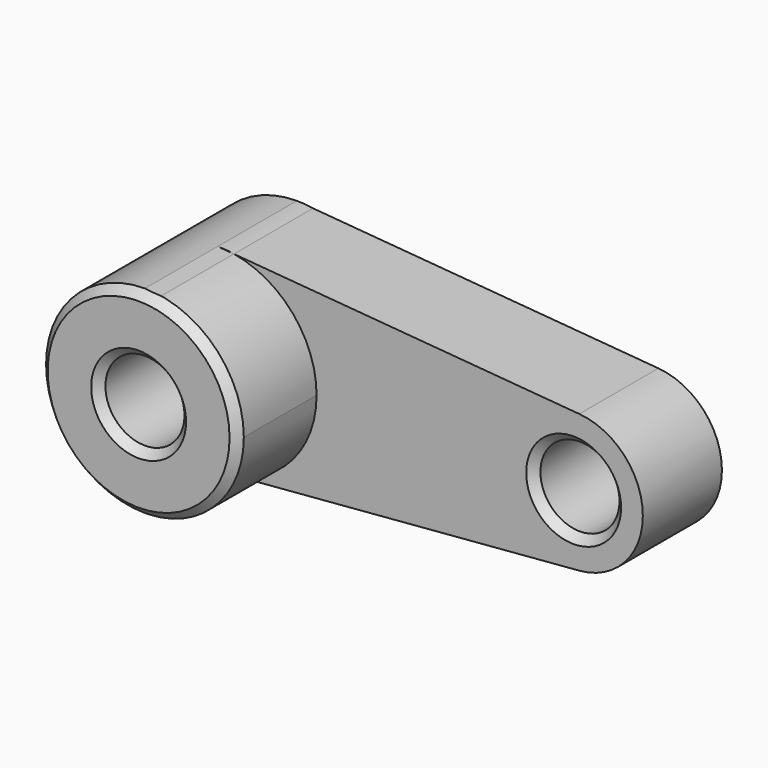
from build123d import *

# Parameters (mm, degrees)
F0_R        = 10
F1_DEPTH    = 25
F2_DEPTH    = 25
F3_T2_ANGLE = 203.6133668192
F3_T8_ANGLE = 184.7022290241


# Not quite as in the source:
# - a fillet or chamfer that OpenCascade refuses, or shapes differently, is made with other operations: its cross-section is extruded or revolved along the edge and cut away or added


with BuildPart() as f1:
    # F0 (on Front) → F1 (new body)
    with BuildSketch(Plane.XZ):
        with BuildLine():
            Line((4.1054428346, 24.6606029758), (0, 25))
            ThreePointArc((0, 25), (-25, 0), (0, -25))
            Line((0, -25), (4.1054428346, -24.6606029758))
            ThreePointArc((4.1054428346, -24.6606029758), (19.0740146648, -16.1611251022), (25, 0))
            ThreePointArc((25, 0), (19.0740146648, 16.1611251022), (4.1054428346, 24.6606029758))
        make_face()
        Circle(F0_R, mode=Mode.SUBTRACT)
        with BuildLine():
            ThreePointArc((4.1054428346, 24.6606029758), (2.0597239626, 24.9150062653), (0, 25))
            Line((0, 25), (4.1054428346, 24.6606029758))
        make_face()
        with BuildLine():
            Line((4.1054428346, -24.6606029758), (0, -25))
            ThreePointArc((0, -25), (2.0597239626, -24.9150062653), (4.1054428346, -24.6606029758))
        make_face()
        with BuildLine():
            Line((91.4418067738, 17.4405043857), (4.1054428346, 24.6606029758))
            ThreePointArc((4.1054428346, 24.6606029758), (19.0740146648, 16.1611251022), (25, 0))
            ThreePointArc((25, 0), (19.0740146648, -16.1611251022), (4.1054428346, -24.6606029758))
            Line((4.1054428346, -24.6606029758), (91.4418067738, -17.4405043857))
            ThreePointArc((91.4418067738, -17.4405043857), (72.5, 0), (91.4418067738, 17.4405043857))
        make_face()
        with BuildLine():
            ThreePointArc((107.5, 0), (102.8740362463, 11.8536572723), (91.4418067738, 17.4405043857))
            ThreePointArc((91.4418067738, 17.4405043857), (72.5, 0), (91.4418067738, -17.4405043857))
            ThreePointArc((91.4418067738, -17.4405043857), (102.8740362463, -11.8536572723), (107.5, 0))
        make_face()
        with Locations((90, 0)):
            Circle(F0_R, mode=Mode.SUBTRACT)
    extrude(amount=-F1_DEPTH)

    # F0 (on Front) → F2 (join)
    with BuildSketch(Plane.XZ):
        with BuildLine():
            Line((4.1054428346, 24.6606029758), (0, 25))
            ThreePointArc((0, 25), (-25, 0), (0, -25))
            Line((0, -25), (4.1054428346, -24.6606029758))
            ThreePointArc((4.1054428346, -24.6606029758), (19.0740146648, -16.1611251022), (25, 0))
            ThreePointArc((25, 0), (19.0740146648, 16.1611251022), (4.1054428346, 24.6606029758))
        make_face()
        Circle(F0_R, mode=Mode.SUBTRACT)
    extrude(amount=F2_DEPTH)

    # F3: chamfer of 2 on 4 edges, made by hand

    # F3_s1 → F3_t2 (revolve, cut)
    with BuildSketch(Plane(origin=(0, 0, 0), x_dir=(0, 1, 0), z_dir=(0.9788435281, 0, -0.2046102329))):
        Polygon((-23, 25), (-25, 23), (-25, 25), align=None)
    revolve(axis=Axis((0, -25, 0), (0, -1, 0)), revolution_arc=F3_T2_ANGLE, mode=Mode.SUBTRACT)

    # F3_s3 → F3_t4 (revolve, cut)
    with BuildSketch(Plane.XY):
        Polygon((102, 0), (100, 2), (100, 0), align=None)
    revolve(axis=Axis((90, 0, 0), (0, -1, 0)), mode=Mode.SUBTRACT)

    # F3_s5 → F3_t6 (revolve, cut)
    with BuildSketch(Plane.XY):
        Polygon((12, -25), (10, -23), (10, -25), align=None)
    revolve(axis=Axis((0, -25, 0), (0, -1, 0)), mode=Mode.SUBTRACT)

    # F3_s7 → F3_t8 (revolve, cut)
    with BuildSketch(Plane(origin=(0, 0, 0), x_dir=(0, 1, 0), z_dir=(-0.9991581953, 0, -0.0410231743))):
        Polygon((-23, -25), (-25, -23), (-25, -25), align=None)
    revolve(axis=Axis((0, -25, 0), (0, 1, 0)), revolution_arc=F3_T8_ANGLE, mode=Mode.SUBTRACT)


solid = f1.part
